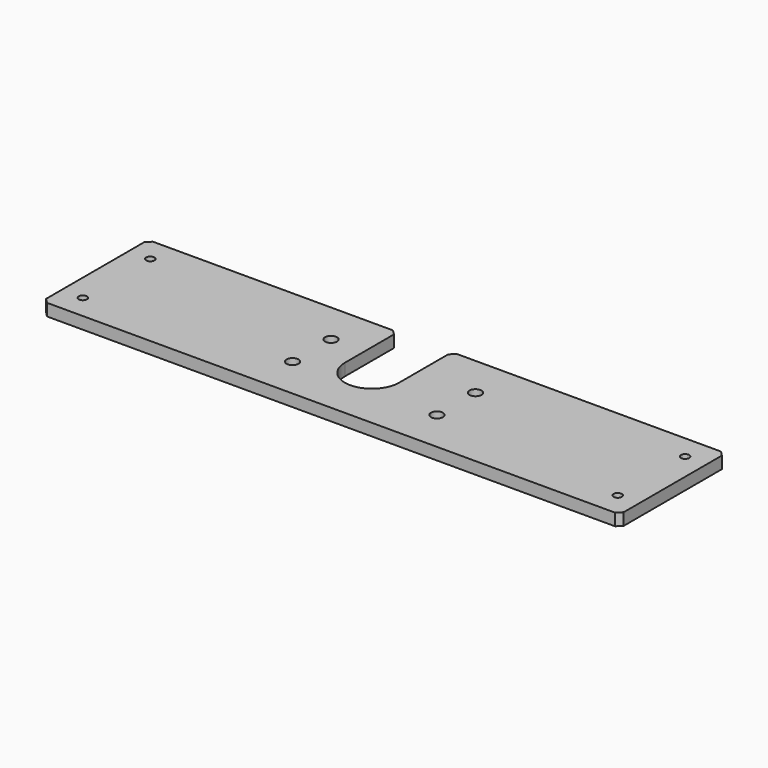
from build123d import *

# Parameters (mm, degrees)
F0_R     = 6.35
F1_DEPTH = 12.7
F2_SIZE  = 5.08
F3_R     = 4.3561
F4_DEPTH = 12.701


with BuildPart() as f1:
    # F0 (on Top) → F1 (new body)
    with BuildSketch(Plane.XY):
        with BuildLine():
            Line((0, 139.7), (0, 0))
            Line((0, 0), (609.6, 0))
            Line((609.6, 0), (609.6, 139.7))
            Line((609.6, 139.7), (333.375, 139.7))
            Line((333.375, 139.7), (320.675, 139.7))
            Line((320.675, 139.7), (320.675, 69.85))
            ThreePointArc((320.675, 69.85), (292.1, 41.275), (263.525, 69.85))
            Line((263.525, 69.85), (263.525, 139.7))
            Line((263.525, 139.7), (0, 139.7))
        make_face()
        with Locations((228.6, 44.45)):
            Circle(F0_R, mode=Mode.SUBTRACT)
        with Locations((381, 44.45)):
            Circle(F0_R, mode=Mode.SUBTRACT)
        with Locations((228.6, 95.25)):
            Circle(F0_R, mode=Mode.SUBTRACT)
        with Locations((381, 95.25)):
            Circle(F0_R, mode=Mode.SUBTRACT)
    extrude(amount=F1_DEPTH)

    # F2
    f2_edges = [f1.edges().sort_by_distance(p)[0] for p in [
        (320.675, 139.7, 6.35),
        (0, 0, 6.35),
        (0, 139.7, 6.35),
        (263.525, 139.7, 6.35),
        (609.6, 139.7, 6.35),
        (609.6, 0, 6.35),
    ]]
    chamfer(f2_edges, length=F2_SIZE)

    # F3 (on face) → F4 (cut, through all)
    with BuildSketch(Plane.XY.offset(12.7)):
        with Locations((22.606, 114.3)):
            Circle(F3_R)
        with Locations((22.606, 25.4)):
            Circle(F3_R)
        with Locations((586.994, 25.4)):
            Circle(F3_R)
        with Locations((586.994, 114.3)):
            Circle(F3_R)
    extrude(amount=-F4_DEPTH, mode=Mode.SUBTRACT)


solid = f1.part
